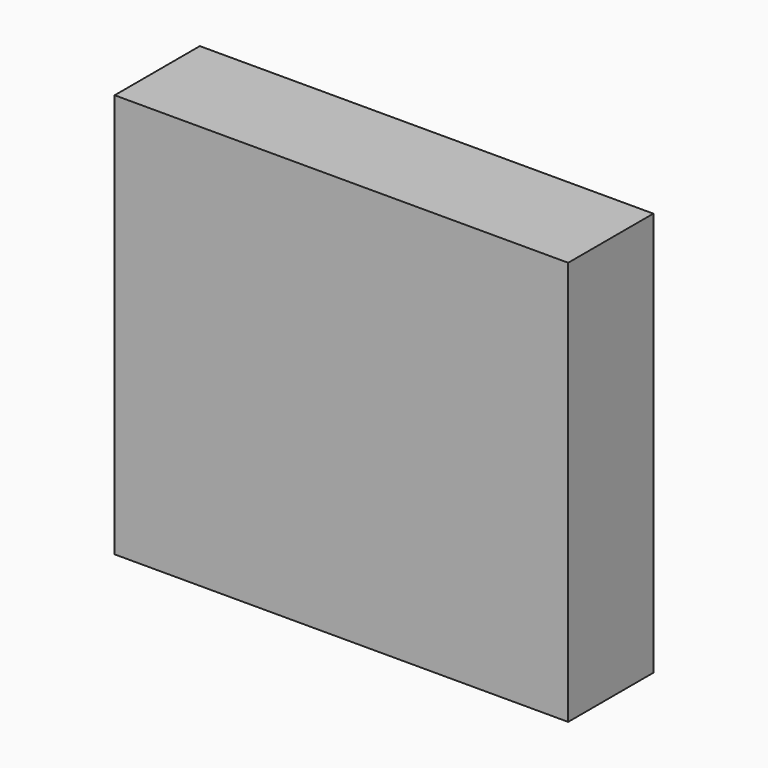
from build123d import *

# Parameters (mm, degrees)
F3_W     = 108.2039736211
F3_H     = 96.4415408671
F0_DEPTH = 25.4


# Not quite as in the source:
# - the program builds the solid bodies; features that only make, move or delete a surface that nothing else refers to are left out


with BuildPart() as f0:
    # F3 (on Front) → F0 (new body)
    with BuildSketch(Plane.XZ):
        with Locations((42.9259706289, 43.0409889668)):
            Rectangle(F3_W, F3_H)
    extrude(amount=F0_DEPTH)


solid = f0.part
